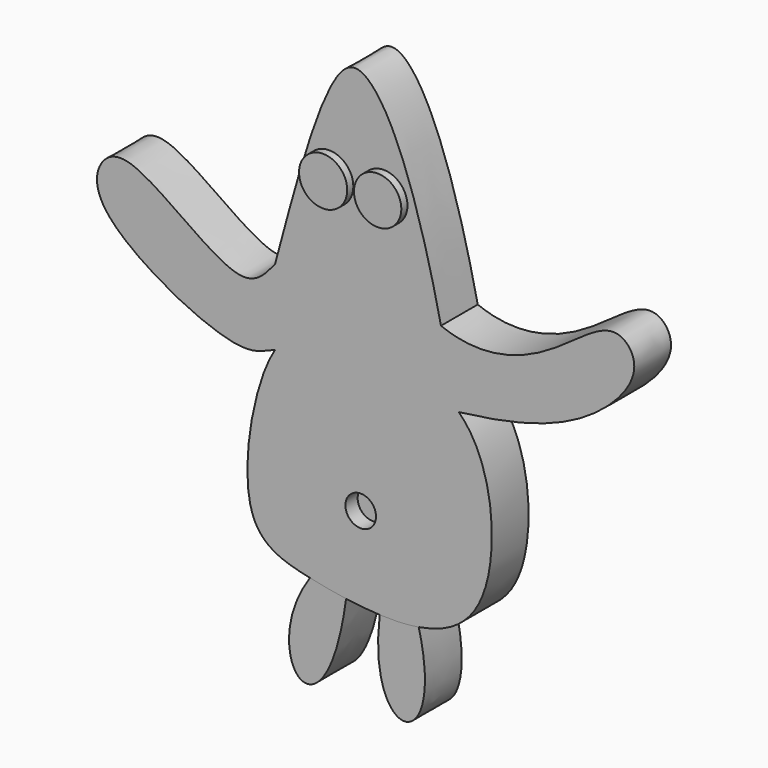
from build123d import *

# Parameters (mm, degrees)
F1_DEPTH = 7.62
F0_R     = 2.54
F0_R_2   = 3.9939806537
F0_R_3   = 3.9284974706
F2_DEPTH = 7.62
F3_DEPTH = 5.08
F4_DEPTH = 8.89


# Not quite as in the source:
# - the program builds the solid bodies; features that only make, move or delete a surface that nothing else refers to are left out


with BuildPart() as f1:
    # F0 (on Front) → F1 (new body)
    with BuildSketch(Plane.XZ):
        with BuildLine():
            add(Edge.make_bspline(
                [(8.3666636462, -14.1454465296), (6.029789649, -33.4373401662), (19.6278417799, -32.8450004155), (14.8436188205, -13.8335144685)],
                knots=[0, 0, 0, 0, 6.4844621936, 6.4844621936, 6.4844621936, 6.4844621936], degree=3))
            add(Edge.make_bspline(
                [(8.3666636462, -14.1454465296), (10.6135470113, -14.2419683118), (12.8138183967, -14.1663312208), (14.8436188205, -13.8335144685)],
                knots=[0.5198636917, 0.5198636917, 0.5198636917, 0.5198636917, 0.5921042973, 0.5921042973, 0.5921042973, 0.5921042973], degree=3))
        make_face()
    extrude(amount=F1_DEPTH)


with BuildPart() as f1b:
    # F0 (on Front) → F1, piece 2 (new body)
    with BuildSketch(Plane.XZ):
        with BuildLine():
            add(Edge.make_bspline(
                [(-3.1972652372, -12.5119319602), (-1.3151625577, -12.9185913113), (0.7131765353, -13.3052102147), (2.7891159978, -13.6040817179)],
                knots=[0.3934029012, 0.3934029012, 0.3934029012, 0.3934029012, 0.4603632064, 0.4603632064, 0.4603632064, 0.4603632064], degree=3))
            add(Edge.make_bspline(
                [(-3.1972652372, -12.5119319602), (-12.462811752, -25.9623099587), (-0.6314517375, -39.1190569146), (2.7891159978, -13.6040817179)],
                knots=[0, 0, 0, 0, 6.0851911542, 6.0851911542, 6.0851911542, 6.0851911542], degree=3))
        make_face()
    extrude(amount=F1_DEPTH)


with BuildPart() as f2:
    # F0 (on Front) → F2 (new body)
    with BuildSketch(Plane.XZ):
        with BuildLine():
            add(Edge.make_bspline(
                [(-8.9937544885, 31.3960482013), (-5.9915025392, 42.6219161305), (-1.6327954119, 58.8866397675), (4.2070541108, 66.1904595846), (11.504848366, 58.3829205052), (16.1555024803, 42.4030038871), (18.5296721756, 31.3615985215)],
                knots=[0, 0, 0, 0, 0.3400171135, 0.4945935455, 0.6631256428, 1, 1, 1, 1], degree=3))
            add(Edge.make_bspline(
                [(-8.9937544885, 31.3960482013), (-10.588841216, 29.4504608313), (-14.7968603022, 23.9793284468), (-32.7647731978, 41.3339309758), (-39.0535280955, 36.4992386423), (-38.4107698736, 27.6223081289), (-14.7737804344, 15.065397303), (-10.4507993177, 18.4069307098), (-8.9937544885, 18.8877706602)],
                knots=[0, 0, 0, 0, 0.1336405217, 0.3698024812, 0.4851626371, 0.6218141221, 0.8764760522, 1, 1, 1, 1], degree=3))
            add(Edge.make_bspline(
                [(-8.9937544885, 18.8877706602), (-12.4212934669, 13.4963097912), (-16.6678709626, -8.8857696906), (-7.6368253061, -11.5526917252), (-3.1972652372, -12.5119319602)],
                knots=[0, 0, 0, 0, 0.2354549315, 0.3934029012, 0.3934029012, 0.3934029012, 0.3934029012], degree=3))
            add(Edge.make_bspline(
                [(-3.1972652372, -12.5119319602), (-1.3151625577, -12.9185913113), (0.7131765353, -13.3052102147), (2.7891159978, -13.6040817179)],
                knots=[0.3934029012, 0.3934029012, 0.3934029012, 0.3934029012, 0.4603632064, 0.4603632064, 0.4603632064, 0.4603632064], degree=3))
            add(Edge.make_bspline(
                [(2.7891159978, -13.6040817179), (4.6337821072, -13.8696569638), (6.5160333844, -14.0659470175), (8.3666636462, -14.1454465296)],
                knots=[0.4603632064, 0.4603632064, 0.4603632064, 0.4603632064, 0.5198636917, 0.5198636917, 0.5198636917, 0.5198636917], degree=3))
            add(Edge.make_bspline(
                [(8.3666636462, -14.1454465296), (10.6135470113, -14.2419683118), (12.8138183967, -14.1663312208), (14.8436188205, -13.8335144685)],
                knots=[0.5198636917, 0.5198636917, 0.5198636917, 0.5198636917, 0.5921042973, 0.5921042973, 0.5921042973, 0.5921042973], degree=3))
            add(Edge.make_bspline(
                [(14.8436188205, -13.8335144685), (19.6484065411, -13.0456962052), (28.8309215091, -7.7291347863), (27.3585564429, 14.128528491), (21.4862455115, 19.7192072701)],
                knots=[0.5921042973, 0.5921042973, 0.5921042973, 0.5921042973, 0.7631067124, 1, 1, 1, 1], degree=3))
            add(Edge.make_bspline(
                [(21.4862455115, 19.7192072701), (29.0866769589, 20.6365127573), (41.8145994621, 23.2385623251), (52.9175854534, 35.024291152), (46.9252690596, 42.3251964725), (36.2782758063, 31.856292713), (24.9791030222, 28.8016016367), (18.5296721756, 31.3615985215)],
                knots=[0, 0, 0, 0, 0.2528275832, 0.4515890066, 0.574683079, 0.7682747861, 1, 1, 1, 1], degree=3))
        make_face()
        with Locations((5.2184173837, 0)):
            Circle(F0_R, mode=Mode.SUBTRACT)
        with Locations((0, 46.9650253654)):
            Circle(F0_R_2, mode=Mode.SUBTRACT)
        with Locations((9.041313082, 47.1084974706)):
            Circle(F0_R_3, mode=Mode.SUBTRACT)
    extrude(amount=F2_DEPTH)

    # F0 (on Front) → F3 (join)
    with BuildSketch(Plane.XZ):
        with Locations((5.2184173837, 0)):
            Circle(F0_R)
    extrude(amount=F3_DEPTH)

    # F0 (on Front) → F4 (join)
    with BuildSketch(Plane.XZ):
        with Locations((0, 46.9650253654)):
            Circle(F0_R_2)
        with Locations((9.041313082, 47.1084974706)):
            Circle(F0_R_3)
    extrude(amount=F4_DEPTH)


solid = Compound([f1.part, f1b.part, f2.part])
